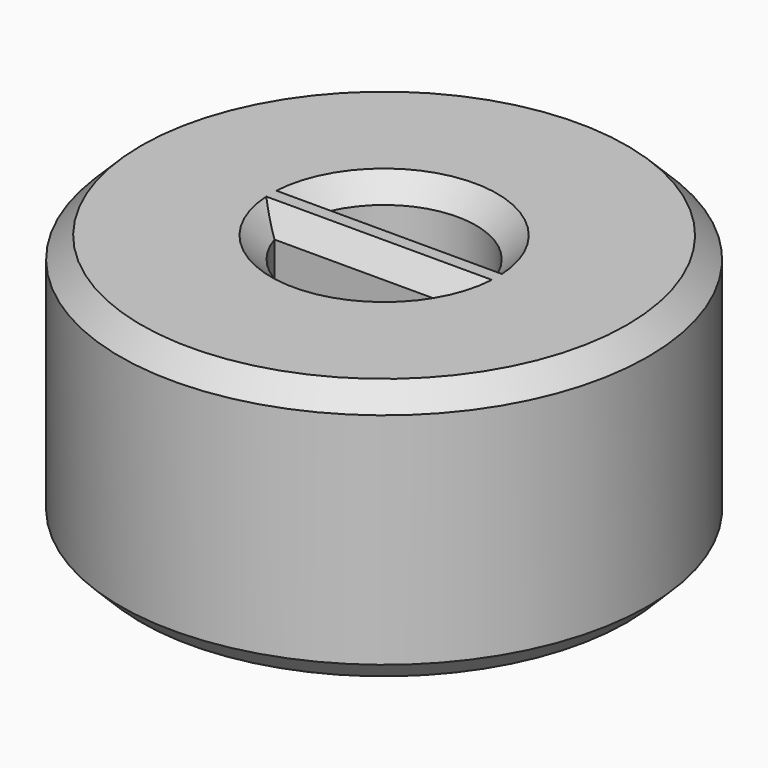
from build123d import *

# Parameters (mm, degrees)
F0_R     = 12.5
F1_DEPTH = 12.4
F2_SIZE  = 1


with BuildPart() as f1:
    # F0 (on Top) → F1 (new body)
    with BuildSketch(Plane.XY):
        Circle(F0_R)
        with BuildLine():
            ThreePointArc((-4.1512046444, 1.3), (0, 4.35), (4.1512046444, 1.3))
            Line((4.1512046444, 1.3), (5, 1.3))
            Line((5, 1.3), (5, -1.3))
            Line((5, -1.3), (4.1512046444, -1.3))
            ThreePointArc((4.1512046444, -1.3), (0, -4.35), (-4.1512046444, -1.3))
            Line((-4.1512046444, -1.3), (-5, -1.3))
            Line((-5, -1.3), (-5, 1.3))
            Line((-5, 1.3), (-4.1512046444, 1.3))
        make_face(mode=Mode.SUBTRACT)
        with BuildLine():
            ThreePointArc((4.1512046444, -1.3), (4.3000139653, -0.657556004), (4.35, 0))
            ThreePointArc((4.35, 0), (4.3000139653, 0.657556004), (4.1512046444, 1.3))
            Line((4.1512046444, 1.3), (-4.1512046444, 1.3))
            ThreePointArc((-4.1512046444, 1.3), (-4.35, 0), (-4.1512046444, -1.3))
            Line((-4.1512046444, -1.3), (4.1512046444, -1.3))
        make_face()
        with BuildLine():
            ThreePointArc((4.1512046444, 1.3), (4.3000139653, 0.657556004), (4.35, 0))
            ThreePointArc((4.35, 0), (4.3000139653, -0.657556004), (4.1512046444, -1.3))
            Line((4.1512046444, -1.3), (5, -1.3))
            Line((5, -1.3), (5, 1.3))
            Line((5, 1.3), (4.1512046444, 1.3))
        make_face()
        with BuildLine():
            ThreePointArc((-4.1512046444, -1.3), (-4.35, 0), (-4.1512046444, 1.3))
            Line((-4.1512046444, 1.3), (-5, 1.3))
            Line((-5, 1.3), (-5, -1.3))
            Line((-5, -1.3), (-4.1512046444, -1.3))
        make_face()
    extrude(amount=F1_DEPTH)

    # F2
    f2_edges = [f1.edges().sort_by_distance(p)[0] for p in [
        (-12.5, 0, 12.4),
        (0, -4.35, 12.4),
        (0, -1.3, 12.4),
        (0, 1.3, 12.4),
        (0, 4.35, 12.4),
        (-12.5, 0, 0),
        (0, 1.3, 0),
        (0, 4.35, 0),
        (0, -1.3, 0),
        (0, -4.35, 0),
    ]]
    chamfer(f2_edges, length=F2_SIZE)


solid = f1.part
